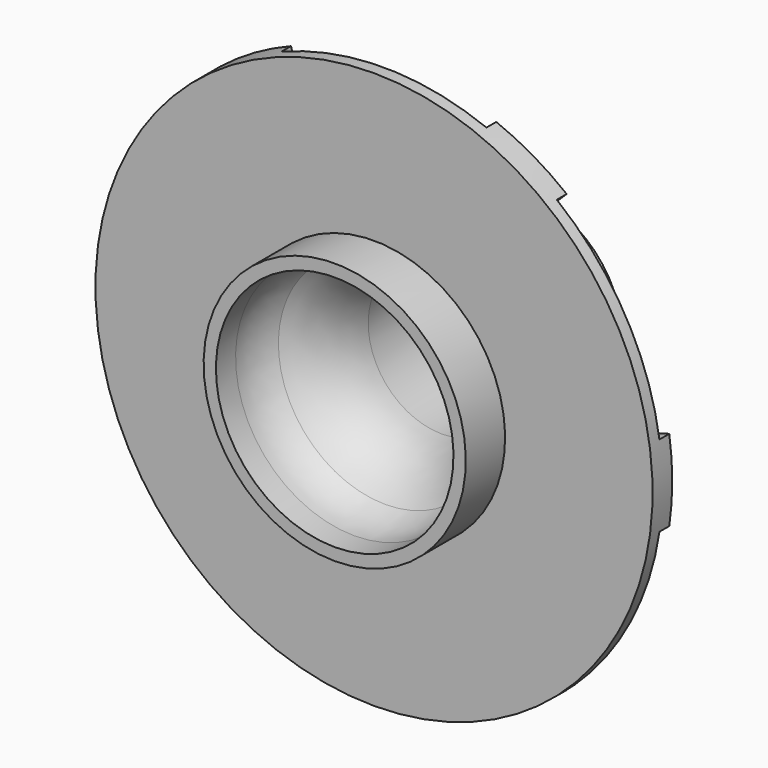
from build123d import *

# Parameters (mm, degrees)
F0_W     = 20
F0_H     = 10
F0_H_2   = 120
F0_W_2   = 83.6363699974
F0_H_3   = 20
F3_DEPTH = 10
F4_DEPTH = 10


with BuildPart() as f1:
    # F0 (on Right) → F1 (revolve)
    with BuildSketch(Plane.YZ):
        with Locations((-54.3666072938, -174.1780357832)):
            Rectangle(F0_W, F0_H)
        with BuildLine():
            ThreePointArc((-12.7470903483, -159.618054612), (-27.8500467267, -166.7357841949), (-44.3666072938, -169.1780357832))
            Line((-44.3666072938, -169.1780357832), (-44.3666072938, -179.1780357832))
            Line((-44.3666072938, -179.1780357832), (-24.3666072938, -179.1780357832))
            ThreePointArc((-24.3666072938, -179.1780357832), (-19.3081292942, -168.9517504843), (-12.7470903483, -159.618054612))
        make_face()
        with Locations((-14.3666072938, -239.1780357832)):
            Rectangle(F0_W, F0_H_2)
        with Locations((86.542492088, -142.5113668702)):
            Rectangle(F0_W_2, F0_H_3)
        with BuildLine():
            ThreePointArc((44.7243070893, -132.5113668702), (12.9527237019, -139.6280506805), (-12.7470903483, -159.618054612))
            ThreePointArc((-12.7470903483, -159.618054612), (-19.3081292942, -168.9517504843), (-24.3666072938, -179.1780357832))
            Line((-24.3666072938, -179.1780357832), (-4.3666072938, -179.1780357832))
            ThreePointArc((-4.3666072938, -179.1780357832), (16.7912213938, -159.6083850702), (44.7243070893, -152.5113668702))
            Line((44.7243070893, -152.5113668702), (44.7243070893, -132.5113668702))
        make_face()
    revolve(axis=Axis((0, 35.6333935665, -72.5113668702), (0, 1, 0)))

    # F2 (on face) → F3 (cut)
    with BuildSketch(Plane(origin=(0, -4.3666072938, 0), x_dir=(-1, 0, 0), z_dir=(0, 1, 0))):
        with BuildLine():
            ThreePointArc((224.2430593698, -105.5693329389), (122.6869341482, -143.3447013267), (140.7505680979, -250.1825698723))
            ThreePointArc((140.7505680979, -250.1825698723), (196.2990934699, -185.8447013267), (224.2430593698, -105.5693329389))
        make_face()
    extrude(amount=-F3_DEPTH, mode=Mode.SUBTRACT)

    # F2 (on face) → F4 (cut)
    with BuildSketch(Plane(origin=(0, -4.3666072938, 0), x_dir=(-1, 0, 0), z_dir=(0, 1, 0))):
        with BuildLine():
            ThreePointArc((-83.4924912719, -283.2405359411), (0, -299.1780357832), (83.4924912719, -283.2405359411))
            ThreePointArc((83.4924912719, -283.2405359411), (0, -214.1780357832), (-83.4924912719, -283.2405359411))
        make_face()
        with BuildLine():
            ThreePointArc((-224.2430593698, -105.5693329389), (-196.2990934699, -185.8447013267), (-140.7505680979, -250.1825698723))
            ThreePointArc((-140.7505680979, -250.1825698723), (-122.6869341482, -143.3447013267), (-224.2430593698, -105.5693329389))
        make_face()
        with BuildLine():
            ThreePointArc((-140.7505680979, 105.159836132), (-196.2990934699, 40.8219675864), (-224.2430593698, -39.4534008014))
            ThreePointArc((-224.2430593698, -39.4534008014), (-122.6869341482, -1.6780324136), (-140.7505680979, 105.159836132))
        make_face()
        with BuildLine():
            ThreePointArc((140.7505680979, 105.159836132), (122.6869341482, -1.6780324136), (224.2430593698, -39.4534008014))
            ThreePointArc((224.2430593698, -39.4534008014), (196.2990934699, 40.8219675864), (140.7505680979, 105.159836132))
        make_face()
        with BuildLine():
            ThreePointArc((83.4924912719, 138.2178022008), (0, 154.1553020429), (-83.4924912719, 138.2178022008))
            ThreePointArc((-83.4924912719, 138.2178022008), (0, 69.1553020429), (83.4924912719, 138.2178022008))
        make_face()
    extrude(amount=-F4_DEPTH, mode=Mode.SUBTRACT)


solid = f1.part
